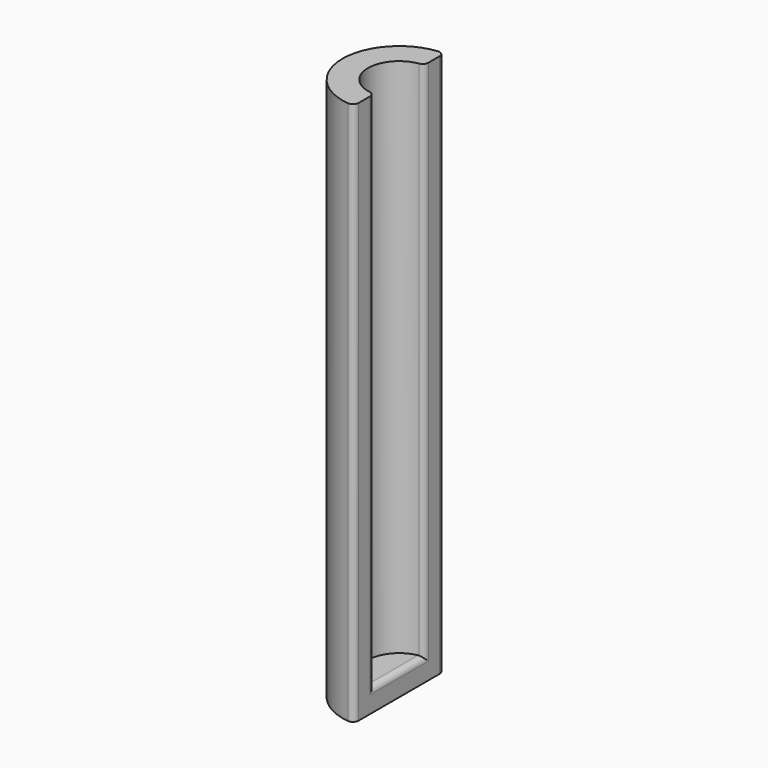
from build123d import *

# Parameters (mm, degrees)
F1_DEPTH = 48
F2_DEPTH = 2
F3_R     = 0.5


with BuildPart() as f1:
    # F0 (on Top) → F1 (new body)
    with BuildSketch(Plane.XY):
        with BuildLine():
            Line((0, 2.75), (0, 5))
            ThreePointArc((0, 5), (-5, 0), (0, -5))
            Line((0, -5), (0, -2.75))
            ThreePointArc((0, -2.75), (-2.75, 0), (0, 2.75))
        make_face()
    extrude(amount=F1_DEPTH)

    # F0 (on Top) → F2 (join)
    with BuildSketch(Plane.XY):
        with BuildLine():
            Line((0, 2.75), (0, 5))
            ThreePointArc((0, 5), (-5, 0), (0, -5))
            Line((0, -5), (0, -2.75))
            ThreePointArc((0, -2.75), (-2.75, 0), (0, 2.75))
        make_face()
        with BuildLine():
            Line((0, -2.75), (0, 2.75))
            ThreePointArc((0, 2.75), (-2.75, 0), (0, -2.75))
        make_face()
    extrude(amount=F2_DEPTH)

    # F3
    f3_edges = [f1.edges().sort_by_distance(p)[0] for p in [
        (0, 2.75, 25),
        (0, -2.75, 25),
        (0, -5, 24),
        (0, 0, 2),
        (0, 5, 24),
    ]]
    fillet(f3_edges, radius=F3_R)


solid = f1.part
